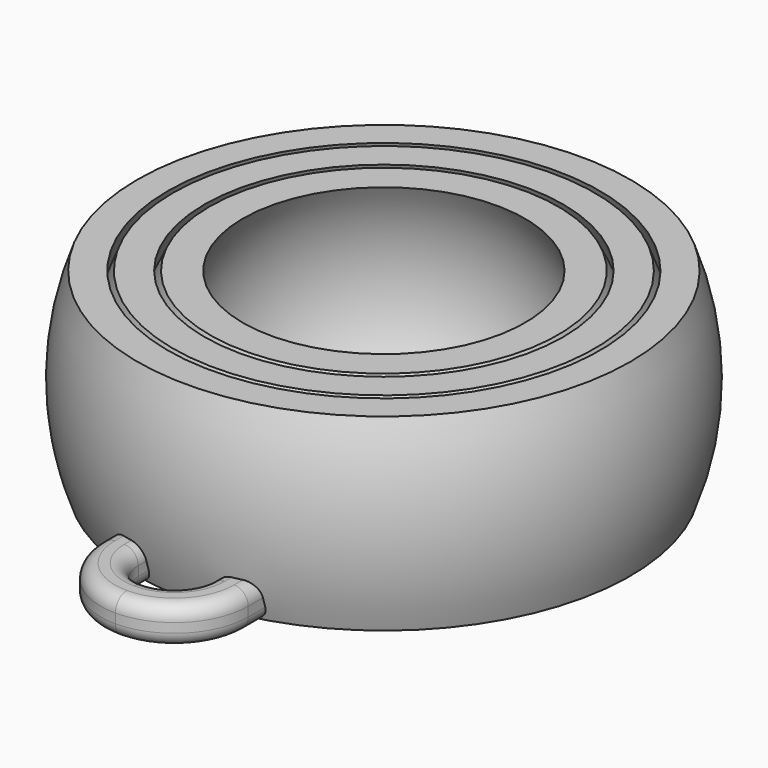
from build123d import *

# Parameters (mm, degrees)
F3_DEPTH = 2
F4_R     = 0.75


with BuildPart() as f1:
    # F0 (on Front) → F1 (revolve)
    with BuildSketch(Plane.XZ):
        with BuildLine():
            ThreePointArc((-11.4564392374, 0), (-12.5, 5), (-11.4564392374, 10))
            Line((-11.4564392374, 10), (-13.0766968306, 10))
            ThreePointArc((-13.0766968306, 10), (-14, 5), (-13.0766968306, 0))
            Line((-13.0766968306, 0), (-11.4564392374, 0))
        make_face()
    revolve(axis=Axis((0, 0, 5), (0, 0, 1)))

    # F2 (on face) → F3 (join)
    with BuildSketch(Plane(origin=(0, 0, 0), x_dir=(1, 0, 0), z_dir=(0, 0, -1))):
        with BuildLine():
            Line((-3.9126477204, 13.8850705698), (-3.9126477204, 12.4776274915))
            ThreePointArc((-3.9126477204, 12.4776274915), (-2.9216532973, 12.7461343948), (-1.9126477204, 12.9360650392))
            Line((-1.9126477204, 12.9360650392), (-1.9126477204, 13.8850705698))
            ThreePointArc((-1.9126477204, 13.8850705698), (-1.3524461731, 15.2375167429), (0, 15.7977182902))
            ThreePointArc((0, 15.7977182902), (1.3524461731, 15.2375167429), (1.9126477204, 13.8850705698))
            Line((1.9126477204, 13.8850705698), (1.9126477204, 12.9360650392))
            ThreePointArc((1.9126477204, 12.9360650392), (2.9216532973, 12.7461343948), (3.9126477204, 12.4776274915))
            Line((3.9126477204, 12.4776274915), (3.9126477204, 13.8850705698))
            ThreePointArc((3.9126477204, 13.8850705698), (2.7666597355, 16.6517303053), (0, 17.7977182902))
            ThreePointArc((0, 17.7977182902), (-2.7666597355, 16.6517303053), (-3.9126477204, 13.8850705698))
        make_face()
    extrude(amount=-F3_DEPTH)

    # F4
    f4_edges = [f1.edges().sort_by_distance(p)[0] for p in [
        (0, -17.797718, 2),
        (0, -15.797718, 2),
        (0, -17.797718, 0),
        (0, -15.797718, 0),
    ]]
    fillet(f4_edges, radius=F4_R)


with BuildPart() as f1b:
    # F0 (on Front) → F1, piece 2 (revolve)
    with BuildSketch(Plane.XZ):
        with BuildLine():
            ThreePointArc((-9.5164331553, 0), (-10.75, 5), (-9.5164331553, 10))
            Line((-9.5164331553, 10), (-11.1831346232, 10))
            ThreePointArc((-11.1831346232, 10), (-12.25, 5), (-11.1831346232, 0))
            Line((-11.1831346232, 0), (-9.5164331553, 0))
        make_face()
    revolve(axis=Axis((0, 0, 5), (0, 0, 1)))


with BuildPart() as f1c:
    # F0 (on Front) → F1, piece 3 (revolve)
    with BuildSketch(Plane.XZ):
        with BuildLine():
            ThreePointArc((-7.4833147735, 0), (-9, 5), (-7.4833147735, 10))
            Line((-7.4833147735, 10), (-9.2330926563, 10))
            ThreePointArc((-9.2330926563, 10), (-10.5, 5), (-9.2330926563, 0))
            Line((-9.2330926563, 0), (-7.4833147735, 0))
        make_face()
    revolve(axis=Axis((0, 0, 5), (0, 0, 1)))


solid = Compound([f1.part, f1b.part, f1c.part])
